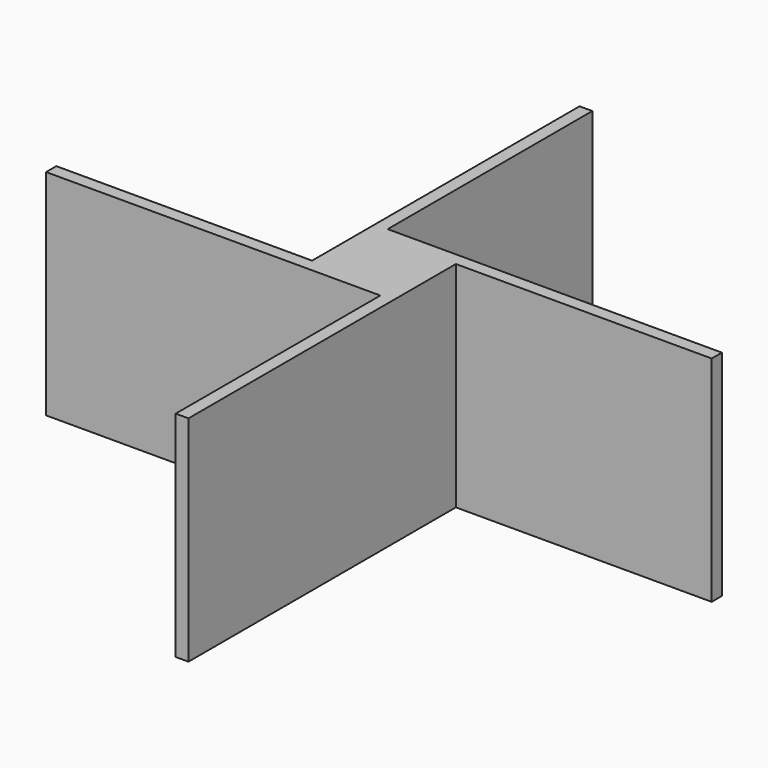
from build123d import *

# Parameters (mm, degrees)
F7_DEPTH = 21.2725
F8_R     = 2.413
F9_DEPTH = 20.0025
F10_R    = 2.413


# Not quite as in the source:
# - a variable given as a bare number and used for a length is read in inches; the dataset says mm whatever the document's units were


with BuildPart() as f7:
    # F6 (on Top) → F7 (new body)
    with BuildSketch(Plane.XY):
        Polygon((-100.2214143808, -23.920097865), (-92.4320810475, -23.920097865), (-92.4320810475, -49.320097865), (-91.1620810475, -49.320097865), (-91.1620810475, -23.920097865), (-91.1620810475, -16.1307645317), (-65.7620810475, -16.1307645317), (-65.7620810475, -14.8607645317), (-91.1620810475, -14.8607645317), (-93.2787477141, -14.8607645317), (-98.9514143808, -14.8607645317), (-98.9514143808, 10.5392354683), (-100.2214143808, 10.5392354683), (-100.2214143808, -14.8607645317), (-100.2214143808, -22.650097865), (-125.6214143808, -22.650097865), (-125.6214143808, -23.920097865), align=None)
    extrude(amount=F7_DEPTH)

    # F8 (on face) → F9 (cut)
    with BuildSketch(Plane(origin=(0, 0, 0), x_dir=(1, 0, 0), z_dir=(0, 0, -1))):
        with Locations((-95.6917477141, 19.3904311984)):
            Circle(F8_R)
    extrude(amount=-F9_DEPTH, mode=Mode.SUBTRACT)

    # F10
    f10_edges = [f7.edges().sort_by_distance(p)[0] for p in [
        (-98.104748, -19.390431, 20.0025),
    ]]
    fillet(f10_edges, radius=F10_R)


solid = f7.part
